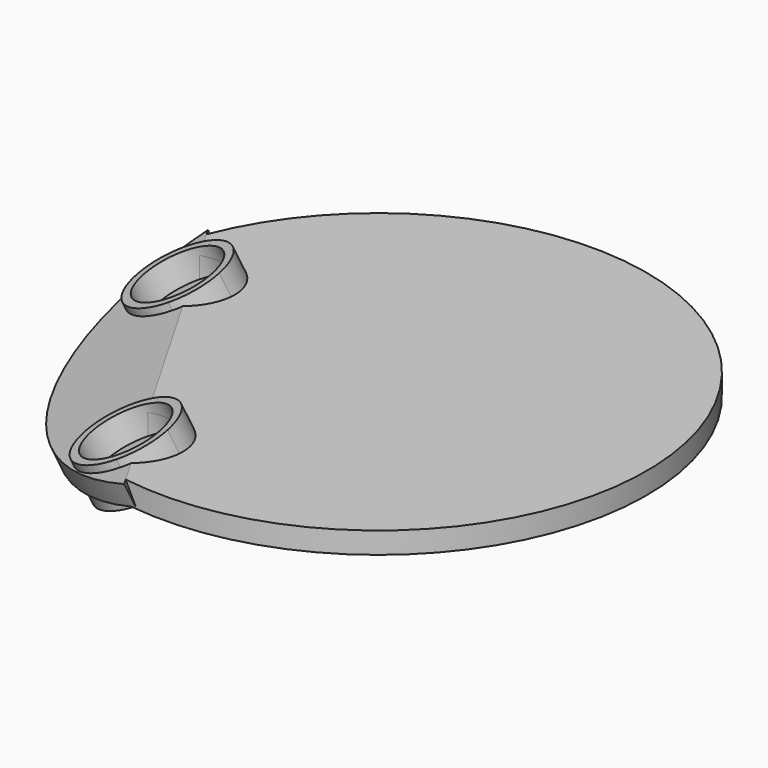
from build123d import *
from build123d import SkipClean  # not in build123d's __all__

# Parameters (mm, degrees)
F2_DEPTH      = 4
F4_DEPTH      = 5
F5_DEPTH      = 45.5098150694
F5_DEPTH_BACK = 23.1317451549
F6_DEPTH      = 3
F9_DEPTH      = 4


with BuildPart() as f2:
    # F0 (on Top) → F2 (new body)
    with BuildSketch(Plane.XY):
        with BuildLine():
            Line((27.041634566, -15.612494996), (39.541634566, 6.0381400986))
            ThreePointArc((39.541634566, 6.0381400986), (34.6410161514, 20), (25, 31.224989992))
            Line((25, 31.224989992), (0, 31.224989992))
            Line((0, 31.224989992), (0, 0))
            Line((0, 0), (27.041634566, -15.612494996))
        make_face()
        with BuildLine():
            ThreePointArc((-14.541634566, -37.2631300906), (0, -40), (14.541634566, -37.2631300906))
            Line((14.541634566, -37.2631300906), (27.041634566, -15.612494996))
            Line((27.041634566, -15.612494996), (0, 0))
            Line((0, 0), (-27.041634566, -15.612494996))
            Line((-27.041634566, -15.612494996), (-14.541634566, -37.2631300906))
        make_face()
        with BuildLine():
            Line((0, 31.224989992), (-25, 31.224989992))
            ThreePointArc((-25, 31.224989992), (-34.6410161514, 20), (-39.541634566, 6.0381400986))
            Line((-39.541634566, 6.0381400986), (-27.041634566, -15.612494996))
            Line((-27.041634566, -15.612494996), (0, 0))
            Line((0, 0), (0, 31.224989992))
        make_face()
        with BuildLine():
            ThreePointArc((14.541634566, -37.2631300906), (33.0277563773, -22.5647359541), (40, 0))
            ThreePointArc((40, 0), (39.8852440298, 3.0277563773), (39.541634566, 6.0381400986))
            Line((39.541634566, 6.0381400986), (27.041634566, -15.612494996))
            Line((27.041634566, -15.612494996), (14.541634566, -37.2631300906))
        make_face()
        with BuildLine():
            Line((0, 31.224989992), (25, 31.224989992))
            ThreePointArc((25, 31.224989992), (0, 40), (-25, 31.224989992))
            Line((-25, 31.224989992), (0, 31.224989992))
        make_face()
        with BuildLine():
            ThreePointArc((39.541634566, 6.0381400986), (39.8852440298, 3.0277563773), (40, 0))
            ThreePointArc((40, 0), (33.0277563773, -22.5647359541), (14.541634566, -37.2631300906))
            ThreePointArc((14.541634566, -37.2631300906), (0, -40), (-14.541634566, -37.2631300906))
            Line((-14.541634566, -37.2631300906), (-7.5160103762, -49.4318681422))
            ThreePointArc((-7.5160103762, -49.4318681422), (32.5898717487, -37.9196553176), (50, 0))
            ThreePointArc((50, 0), (9.2638291816, 49.1343206821), (-46.5672587557, 18.2068781502))
            Line((-46.5672587557, 18.2068781502), (-39.541634566, 6.0381400986))
            ThreePointArc((-39.541634566, 6.0381400986), (-34.6410161514, 20), (-25, 31.224989992))
            ThreePointArc((-25, 31.224989992), (0, 40), (25, 31.224989992))
            ThreePointArc((25, 31.224989992), (34.6410161514, 20), (39.541634566, 6.0381400986))
        make_face()
    extrude(amount=F2_DEPTH)

    # F3 (on line) → F4 (join)
    with BuildSketch(Plane(origin=(-4.8298034606, -2.7884883281, 11.9598650349), x_dir=(0.9306155778, -0.0831049393, 0.3564382351), z_dir=(0.3659981508, 0.2113091309, -0.906307787))):
        with BuildLine():
            ThreePointArc((-41.3294511967, -12.2059585244), (-43.6253957362, -1.8508323218), (-33.2702695336, 0.4451122176))
            Line((-33.2702695336, 0.4451122176), (-32.4643513672, 1.7102192918))
            ThreePointArc((-32.4643513672, 1.7102192918), (-44.8905028104, -1.0449141555), (-42.135369363, -13.4710655987))
            Line((-42.135369363, -13.4710655986), (-41.3294511967, -12.2059585244))
        make_face()
        with BuildLine():
            Line((-32.4643513672, 1.7102192918), (-33.2702695336, 0.4451122176))
            ThreePointArc((-33.2702695336, 0.4451122176), (-30.724454247, -2.2729261844), (-29.7998603651, -5.8804231534))
            ThreePointArc((-29.7998603651, -5.8804231534), (-33.6923633961, -12.4558292716), (-41.3294511967, -12.2059585244))
            Line((-41.3294511967, -12.2059585244), (-42.135369363, -13.4710655986))
            ThreePointArc((-42.135369363, -13.4710655987), (-32.9708640023, -13.7709104952), (-28.2998603651, -5.8804231534))
            ThreePointArc((-28.2998603651, -5.8804231534), (-29.4093730234, -1.5514267906), (-32.4643513672, 1.7102192918))
        make_face()
        with BuildLine():
            ThreePointArc((-5.6004124901, 43.8804550986), (-18.0265639332, 41.1253216513), (-15.2714304859, 28.6991702082))
            Line((-15.2714304859, 28.6991702082), (-14.4655123195, 29.9642772824))
            ThreePointArc((-14.4655123195, 29.9642772824), (-16.761456859, 40.319403485), (-6.4063306564, 42.6153480244))
            Line((-6.4063306564, 42.6153480244), (-5.6004124901, 43.8804550986))
        make_face()
        with BuildLine():
            Line((-14.4655123195, 29.9642772824), (-15.2714304859, 28.6991702082))
            ThreePointArc((-15.2714304859, 28.6991702082), (-6.1069251251, 28.3993253116), (-1.435921488, 36.2898126534))
            ThreePointArc((-1.435921488, 36.2898126534), (-2.5454341462, 40.6188090162), (-5.6004124901, 43.8804550986))
            Line((-5.6004124901, 43.8804550986), (-6.4063306564, 42.6153480244))
            ThreePointArc((-6.4063306564, 42.6153480244), (-3.8605153698, 39.8973096224), (-2.935921488, 36.2898126534))
            ThreePointArc((-2.935921488, 36.2898126534), (-6.8284245189, 29.7144065353), (-14.4655123195, 29.9642772824))
        make_face()
    extrude(amount=-F4_DEPTH)

    # F3 (on line) → F5 (cut, two sides)
    with BuildSketch(Plane(origin=(-4.8298034606, -2.7884883281, 11.9598650349), x_dir=(0.9306155778, -0.0831049393, 0.3564382351), z_dir=(0.3659981508, 0.2113091309, -0.906307787))) as f5_sk:
        with BuildLine():
            Line((-41.3294511967, -12.2059585244), (-37.2998603651, -5.8804231534))
            Line((-37.2998603651, -5.8804231534), (-33.2702695336, 0.4451122176))
            ThreePointArc((-33.2702695336, 0.4451122176), (-43.6253957362, -1.8508323218), (-41.3294511967, -12.2059585244))
        make_face()
        with BuildLine():
            Line((-33.2702695336, 0.4451122176), (-37.2998603651, -5.8804231534))
            Line((-37.2998603651, -5.8804231534), (-41.3294511967, -12.2059585244))
            ThreePointArc((-41.3294511967, -12.2059585244), (-33.6923633961, -12.4558292716), (-29.7998603651, -5.8804231534))
            ThreePointArc((-29.7998603651, -5.8804231534), (-30.724454247, -2.2729261844), (-33.2702695336, 0.4451122176))
        make_face()
        with BuildLine():
            ThreePointArc((-6.4063306564, 42.6153480244), (-16.761456859, 40.319403485), (-14.4655123195, 29.9642772824))
            Line((-14.4655123195, 29.9642772824), (-10.435921488, 36.2898126534))
            Line((-10.435921488, 36.2898126534), (-6.4063306564, 42.6153480244))
        make_face()
        with BuildLine():
            Line((-10.435921488, 36.2898126534), (-14.4655123195, 29.9642772824))
            ThreePointArc((-14.4655123195, 29.9642772824), (-6.8284245189, 29.7144065353), (-2.935921488, 36.2898126534))
            ThreePointArc((-2.935921488, 36.2898126534), (-3.8605153698, 39.8973096224), (-6.4063306564, 42.6153480244))
            Line((-6.4063306564, 42.6153480244), (-10.435921488, 36.2898126534))
        make_face()
    with SkipClean():  # cleaning this boolean's faces spoils the solid; the shape is the same uncleaned
        extrude(amount=F5_DEPTH, mode=Mode.SUBTRACT)
        extrude(f5_sk.sketch, amount=-F5_DEPTH_BACK, mode=Mode.SUBTRACT)

    # F3 (on line) → F6 (join)
    with BuildSketch(Plane(origin=(-4.8298034606, -2.7884883281, 11.9598650349), x_dir=(0.9306155778, -0.0831049393, 0.3564382351), z_dir=(0.3659981508, 0.2113091309, -0.906307787))):
        with BuildLine():
            ThreePointArc((-41.3294511967, -12.2059585244), (-43.6253957362, -1.8508323218), (-33.2702695336, 0.4451122176))
            Line((-33.2702695336, 0.4451122176), (-32.4643513672, 1.7102192918))
            ThreePointArc((-32.4643513672, 1.7102192918), (-44.8905028104, -1.0449141555), (-42.135369363, -13.4710655987))
            Line((-42.135369363, -13.4710655986), (-41.3294511967, -12.2059585244))
        make_face()
        with BuildLine():
            Line((-32.4643513672, 1.7102192918), (-33.2702695336, 0.4451122176))
            ThreePointArc((-33.2702695336, 0.4451122176), (-30.724454247, -2.2729261844), (-29.7998603651, -5.8804231534))
            ThreePointArc((-29.7998603651, -5.8804231534), (-33.6923633961, -12.4558292716), (-41.3294511967, -12.2059585244))
            Line((-41.3294511967, -12.2059585244), (-42.135369363, -13.4710655986))
            ThreePointArc((-42.135369363, -13.4710655987), (-32.9708640023, -13.7709104952), (-28.2998603651, -5.8804231534))
            ThreePointArc((-28.2998603651, -5.8804231534), (-29.4093730234, -1.5514267906), (-32.4643513672, 1.7102192918))
        make_face()
        with BuildLine():
            Line((-41.3294511967, -12.2059585244), (-37.2998603651, -5.8804231534))
            Line((-37.2998603651, -5.8804231534), (-33.2702695336, 0.4451122176))
            ThreePointArc((-33.2702695336, 0.4451122176), (-43.6253957362, -1.8508323218), (-41.3294511967, -12.2059585244))
        make_face()
        with BuildLine():
            Line((-33.2702695336, 0.4451122176), (-37.2998603651, -5.8804231534))
            Line((-37.2998603651, -5.8804231534), (-41.3294511967, -12.2059585244))
            ThreePointArc((-41.3294511967, -12.2059585244), (-33.6923633961, -12.4558292716), (-29.7998603651, -5.8804231534))
            ThreePointArc((-29.7998603651, -5.8804231534), (-30.724454247, -2.2729261844), (-33.2702695336, 0.4451122176))
        make_face()
        with BuildLine():
            ThreePointArc((-5.6004124901, 43.8804550986), (-18.0265639332, 41.1253216513), (-15.2714304859, 28.6991702082))
            Line((-15.2714304859, 28.6991702082), (-14.4655123195, 29.9642772824))
            ThreePointArc((-14.4655123195, 29.9642772824), (-16.761456859, 40.319403485), (-6.4063306564, 42.6153480244))
            Line((-6.4063306564, 42.6153480244), (-5.6004124901, 43.8804550986))
        make_face()
        with BuildLine():
            Line((-14.4655123195, 29.9642772824), (-15.2714304859, 28.6991702082))
            ThreePointArc((-15.2714304859, 28.6991702082), (-6.1069251251, 28.3993253116), (-1.435921488, 36.2898126534))
            ThreePointArc((-1.435921488, 36.2898126534), (-2.5454341462, 40.6188090162), (-5.6004124901, 43.8804550986))
            Line((-5.6004124901, 43.8804550986), (-6.4063306564, 42.6153480244))
            ThreePointArc((-6.4063306564, 42.6153480244), (-3.8605153698, 39.8973096224), (-2.935921488, 36.2898126534))
            ThreePointArc((-2.935921488, 36.2898126534), (-6.8284245189, 29.7144065353), (-14.4655123195, 29.9642772824))
        make_face()
        with BuildLine():
            ThreePointArc((-6.4063306564, 42.6153480244), (-16.761456859, 40.319403485), (-14.4655123195, 29.9642772824))
            Line((-14.4655123195, 29.9642772824), (-10.435921488, 36.2898126534))
            Line((-10.435921488, 36.2898126534), (-6.4063306564, 42.6153480244))
        make_face()
        with BuildLine():
            Line((-10.435921488, 36.2898126534), (-14.4655123195, 29.9642772824))
            ThreePointArc((-14.4655123195, 29.9642772824), (-6.8284245189, 29.7144065353), (-2.935921488, 36.2898126534))
            ThreePointArc((-2.935921488, 36.2898126534), (-3.8605153698, 39.8973096224), (-6.4063306564, 42.6153480244))
            Line((-6.4063306564, 42.6153480244), (-10.435921488, 36.2898126534))
        make_face()
    with SkipClean():  # cleaning this boolean's faces spoils the solid; the shape is the same uncleaned
        extrude(amount=F6_DEPTH)

    # F8 (on offset) → F9 (join)
    with BuildSketch(Plane(origin=(-6.1473968034, -3.5492011993, 15.2225730682), x_dir=(0.9306155778, -0.0831049393, 0.3564382351), z_dir=(0.3659981508, 0.2113091309, -0.906307787))):
        with BuildLine():
            ThreePointArc((-40.62355156, -14.2442187536), (-44.8905028104, -1.0449141555), (-31.1246632897, 0.6668618625))
            Line((-31.1246632897, 0.6668618625), (-13.7596126828, 27.9260170532))
            ThreePointArc((-13.7596126828, 27.9260170532), (-18.0265639332, 41.1253216513), (-4.2607244125, 42.8370976693))
            Line((-4.2607244125, 42.8370976693), (-1.4607309953, 47.2324465122))
            Line((-1.4607309953, 47.2324465122), (-0.697246957, 48.4309417171))
            add(Edge.make_bspline(
                [(-0.697246957, 48.4309417171), (-65.0877492303, 41.4632093827), (-44.1870290155, -19.8380628014)],
                knots=[3.7691820168, 3.7691820168, 3.7691820168, 5.655595944, 5.655595944, 5.655595944], degree=2, weights=[1, 0.5871951872, 1]))
            Line((-44.1870290155, -19.8380628014), (-40.62355156, -14.2442187536))
        make_face()
    extrude(amount=F9_DEPTH)


solid = f2.part
